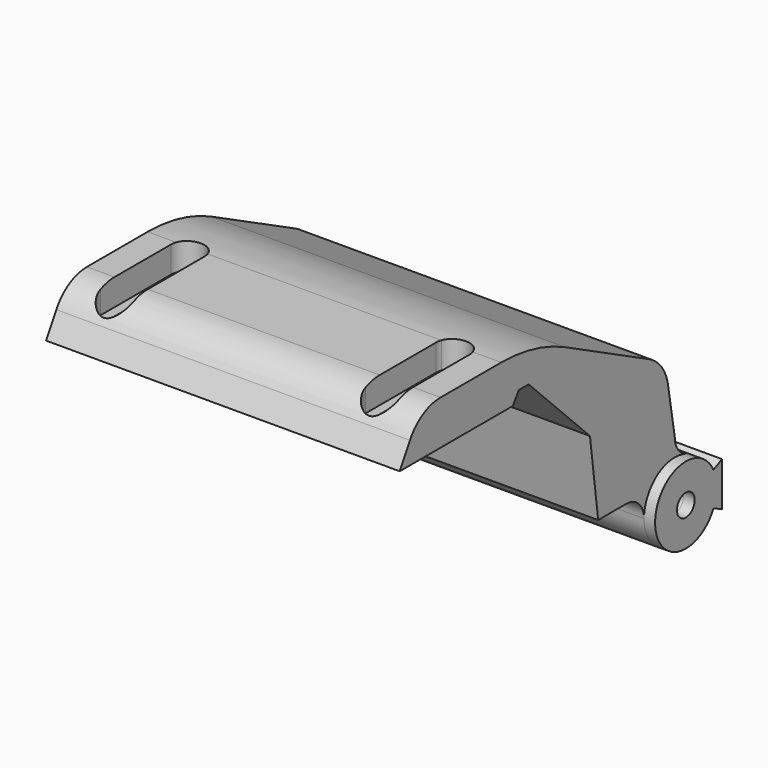
from build123d import *

# Parameters (mm, degrees)
F3_DEPTH      = 50.8
F4_R          = 3.175
F5_DEPTH      = 50.8
F5_DEPTH_BACK = 50.8
F6_R          = 50.8
F7_R          = 12.7
F9_DEPTH      = 12.7
F11_DEPTH     = 7.62
F12_R         = 3.175
F13_DEPTH     = 53.975


# Not quite as in the source:
# - the program builds the solid bodies; features that only make, move or delete a surface that nothing else refers to are left out


with BuildPart() as f3:
    # F2 (on Right) → F3 (new body, symmetric)
    with BuildSketch(Plane.YZ):
        with BuildLine():
            Line((-98.3398951496, 12.7), (-105.6722435683, 0))
            Line((-105.6722435683, 0), (-65.0322435683, 0))
            Line((-65.0322435683, 0), (-62.8906790273, 3.175))
            Line((-62.8906790273, 3.175), (-59.3727790273, 3.175))
            Line((-59.3727790273, 3.175), (-37.3531910185, -18.8445880089))
            Line((-37.3531910185, -18.8445880089), (-34.3958851866, -41.307555944))
            Line((-34.3958851866, -41.307555944), (-21.6958851866, -41.307555944))
            ThreePointArc((-21.6958851866, -41.307555944), (-15.7538496208, -34.2048736472), (-6.8837446161, -31.5445880089))
            Line((-6.8837446161, -31.5445880089), (-10.3898009598, -10.9572655931))
            Line((-10.3898009598, -10.9572655931), (-57.0648951496, 12.7))
            Line((-57.0648951496, 12.7), (-98.3398951496, 12.7))
        make_face()
    extrude(amount=F3_DEPTH, both=True)

    # F4 (on Right) → F5 (join, two sides)
    with BuildSketch(Plane.YZ) as f5_sk:
        with BuildLine():
            Line((-6.8837446161, -31.4737667411), (-6.8837446161, -31.5445880089))
            ThreePointArc((-6.8837446161, -31.5445880089), (-15.7538496208, -34.2048736472), (-21.6958851866, -41.307555944))
            Line((-21.6958851866, -41.307555944), (-24.273218614, -41.307555944))
            ThreePointArc((-24.273218614, -41.307555944), (-19.7824672698, -43.1680512537), (-17.9232188588, -47.6593189789))
            ThreePointArc((-17.9232188588, -47.6593189789), (-0.665383222, -56.7838960892), (-2.8525323178, -37.3852575509))
            ThreePointArc((-2.8525323178, -37.3852575509), (-5.7800195758, -35.0513495908), (-6.8837446161, -31.4737667411))
        make_face()
        with Locations((-6.8837446161, -47.6623840148)):
            Circle(F4_R, mode=Mode.SUBTRACT)
    extrude(amount=F5_DEPTH)
    extrude(f5_sk.sketch, amount=-F5_DEPTH_BACK)

    # F6
    f6_edges = [f3.edges().sort_by_distance(p)[0] for p in [
        (0, -57.064895, 12.7),
    ]]
    fillet(f6_edges, radius=F6_R)

    # F7
    f7_edges = [f3.edges().sort_by_distance(p)[0] for p in [
        (0, -98.339895, 12.7),
        (0, -10.389801, -10.957266),
    ]]
    fillet(f7_edges, radius=F7_R)

    # F8 (on face) → F9 (cut, through all)
    with BuildSketch(Plane(origin=(0, 0, 0), x_dir=(1, 0, 0), z_dir=(0, 0, -1))):
        with BuildLine():
            Line((36.115625, 96.1236006856), (36.115625, 70.7236006856))
            ThreePointArc((36.115625, 70.7236006856), (38.1001408337, 68.7392256906), (40.08437498, 70.7238823529))
            Line((40.08437498, 70.7238823529), (40.0807866095, 96.0043172068))
            Line((40.0807866095, 96.0043172068), (40.0807526669, 96.2434464755))
            ThreePointArc((40.0807526669, 96.2434464755), (38.0400497401, 98.1070698956), (36.115625, 96.1236006856))
        make_face()
        with BuildLine():
            Line((-40.0807866095, 96.0043172068), (-40.08437498, 70.7238823529))
            ThreePointArc((-40.08437498, 70.7238823529), (-38.1001408337, 68.7392256906), (-36.115625, 70.7236006856))
            Line((-36.115625, 70.7236006856), (-36.115625, 96.1236006856))
            ThreePointArc((-36.115625, 96.1236006856), (-38.0400497401, 98.1070698956), (-40.0807526669, 96.2434464755))
            Line((-40.0807526669, 96.2434464755), (-40.0807866095, 96.0043172068))
        make_face()
    extrude(amount=-F9_DEPTH, mode=Mode.SUBTRACT)

    # F10 (on face) → F11 (cut)
    with BuildSketch(Plane.XY.offset(12.7)):
        with BuildLine():
            Line((-42.8625, -70.7236006856), (-42.8625, -96.1236006856))
            ThreePointArc((-42.8625, -96.1236006856), (-38.1, -100.8861006856), (-33.3375, -96.1236006856))
            Line((-33.3375, -96.1236006856), (-33.3375, -91.0075467309))
            Line((-33.3375, -91.0075467309), (-36.115625, -91.0075467309))
            Line((-36.115625, -91.0075467309), (-36.115625, -70.7236006856))
            ThreePointArc((-36.115625, -70.7236006856), (-36.30144514, -69.8851827968), (-36.8241045528, -69.2037865692))
            Line((-36.8241045528, -69.2037865692), (-33.5865122907, -69.2037865692))
            ThreePointArc((-33.5865122907, -69.2037865692), (-38.870039296, -66.0237660361), (-42.8625, -70.7236006856))
        make_face()
        with BuildLine():
            Line((-36.115625, -91.0075467309), (-33.3375, -91.0075467309))
            Line((-33.3375, -91.0075467309), (-33.3375, -70.7236006856))
            ThreePointArc((-33.3375, -70.7236006856), (-33.4001653505, -69.9535613896), (-33.5865122907, -69.2037865692))
            Line((-33.5865122907, -69.2037865692), (-36.8241045528, -69.2037865692))
            ThreePointArc((-36.8241045528, -69.2037865692), (-36.30144514, -69.8851827968), (-36.115625, -70.7236006856))
            Line((-36.115625, -70.7236006856), (-36.115625, -91.0075467309))
        make_face()
        with BuildLine():
            Line((36.115625, -91.0075467309), (33.3375, -91.0075467309))
            Line((33.3375, -91.0075467309), (33.3375, -96.1236006856))
            ThreePointArc((33.3375, -96.1236006856), (38.1, -100.8861006856), (42.8625, -96.1236006856))
            Line((42.8625, -96.1236006856), (42.8625, -70.7236006856))
            ThreePointArc((42.8625, -70.7236006856), (38.870039296, -66.0237660361), (33.5865122907, -69.2037865692))
            Line((33.5865122907, -69.2037865692), (36.8241045528, -69.2037865692))
            ThreePointArc((36.8241045528, -69.2037865692), (36.30144514, -69.8851827968), (36.115625, -70.7236006856))
            Line((36.115625, -70.7236006856), (36.115625, -91.0075467309))
        make_face()
        with BuildLine():
            Line((33.3375, -70.7236006856), (33.3375, -91.0075467309))
            Line((33.3375, -91.0075467309), (36.115625, -91.0075467309))
            Line((36.115625, -91.0075467309), (36.115625, -70.7236006856))
            ThreePointArc((36.115625, -70.7236006856), (36.30144514, -69.8851827968), (36.8241045528, -69.2037865692))
            Line((36.8241045528, -69.2037865692), (33.5865122907, -69.2037865692))
            ThreePointArc((33.5865122907, -69.2037865692), (33.4001653505, -69.9535613896), (33.3375, -70.7236006856))
        make_face()
    extrude(amount=-F11_DEPTH, mode=Mode.SUBTRACT)


with BuildPart() as f13:
    # F12 (on Right) → F13 (new body, symmetric)
    with BuildSketch(Plane.YZ):
        with BuildLine():
            ThreePointArc((3.0300645432, -42.8058019962), (-17.9232192843, -47.6623840148), (3.0300645432, -52.5189660334))
            Line((3.0300645432, -52.5189660334), (6.0785996665, -54.0123840148))
            Line((6.0785996665, -54.0123840148), (6.0785996665, -41.3123840148))
            Line((6.0785996665, -41.3123840148), (3.0300645432, -42.8058019962))
        make_face()
        with Locations((-6.8837446161, -47.6623840148)):
            Circle(F12_R, mode=Mode.SUBTRACT)
    extrude(amount=F13_DEPTH, both=True)

    # F14: cut F3
    add(f3.part, mode=Mode.SUBTRACT)


solid = Compound([f3.part, f13.part])
